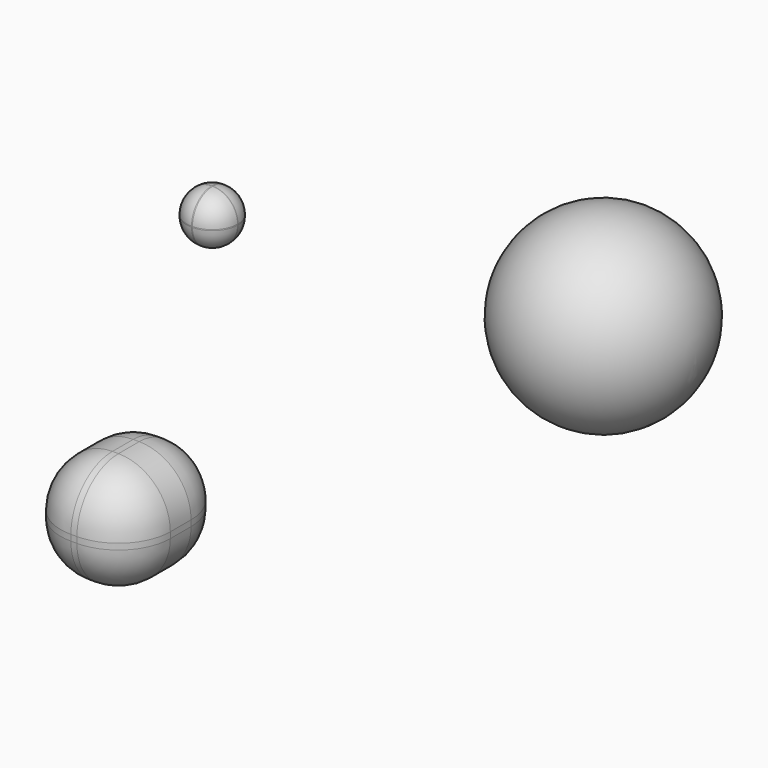
from build123d import *

# Parameters (mm, degrees)
F1_W     = 21.5005669743
F1_H     = 21.5005669743
F2_DEPTH = 25.4
F3_R     = 10.16
F6_W     = 9.9950358272
F6_H     = 9.9950358272
F7_DEPTH = 4.95
F8_R     = 4.9


# Not quite as in the source:
# - ends of sketch curves that miss each other by under 0.0002 mm in the source are joined


with BuildPart() as f2:
    # F1 (on Front) → F2 (new body)
    with BuildSketch(Plane.XZ):
        with Locations((-114.0103889629, -17.3241058365)):
            Rectangle(F1_W, F1_H)
    extrude(amount=F2_DEPTH)

    # F3
    f3_edges = [f2.edges().sort_by_distance(p)[0] for p in [
        (-103.260105, -12.7, -28.074389),
        (-114.010389, -25.4, -28.074389),
        (-124.760672, -12.7, -28.074389),
        (-114.010389, 0, -28.074389),
        (-124.760672, -25.4, -17.324106),
        (-103.260105, -25.4, -17.324106),
        (-114.010389, -25.4, -6.573822),
        (-124.760672, -12.7, -6.573822),
        (-103.260105, -12.7, -6.573822),
        (-114.010389, 0, -6.573822),
        (-124.760672, 0, -17.324106),
        (-103.260105, 0, -17.324106),
    ]]
    fillet(f3_edges, radius=F3_R)


with BuildPart() as f5:
    # F4 (on Front) → F5 (revolve)
    with BuildSketch(Plane.XZ):
        with BuildLine():
            ThreePointArc((-48.8007047402, 37.8541760147), (-30.6370421313, 19.6905134058), (-12.4733795224, 37.8541760147))
            Line((-12.4733795224, 37.8541760147), (-48.8007047402, 37.8541760147))
        make_face()
    revolve(axis=Axis((-30.6370421313, 0, 37.8541760147), (-1, 0, 0)))


with BuildPart() as f7:
    # F6 (on Front) → F7 (new body, symmetric)
    with BuildSketch(Plane.XZ):
        with Locations((-107.2410680354, 30.3790532053)):
            Rectangle(F6_W, F6_H)
    extrude(amount=F7_DEPTH, both=True)

    # F8
    f8_edges = [f7.edges().sort_by_distance(p)[0] for p in [
        (-112.238586, 0, 35.376571),
        (-112.238586, 4.95, 30.379053),
        (-112.238586, 0, 25.381535),
        (-112.238586, -4.95, 30.379053),
        (-102.24355, 4.95, 30.379053),
        (-102.24355, 0, 35.376571),
        (-102.24355, -4.95, 30.379053),
        (-102.24355, 0, 25.381535),
        (-107.241068, 4.95, 35.376571),
        (-107.241068, 4.95, 25.381535),
        (-107.241068, -4.95, 35.376571),
        (-107.241068, -4.95, 25.381535),
    ]]
    fillet(f8_edges, radius=F8_R)


solid = Compound([f2.part, f5.part, f7.part])
